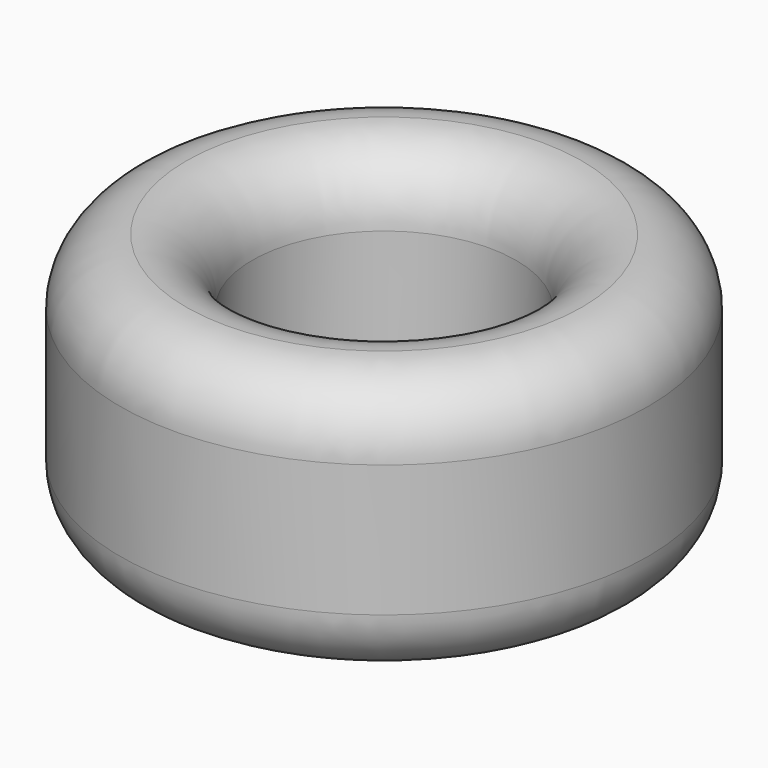
from build123d import *

# Parameters (mm, degrees)
F0_R     = 5.08
F0_R_2   = 2.54
F1_DEPTH = 5.08
F2_R     = 1.26999


# Not quite as in the source:
# - a fillet or chamfer is up to 0.001 mm smaller than in the source, because OpenCascade refuses the exact size


with BuildPart() as f1:
    # F0 (on Top) → F1 (new body)
    with BuildSketch(Plane.XY):
        Circle(F0_R)
        Circle(F0_R_2, mode=Mode.SUBTRACT)
    extrude(amount=F1_DEPTH)

    # F2 (radius 1.27 in the source; OpenCascade refuses exactly that, so slightly less here)
    f2_edges = [f1.edges().sort_by_distance(p)[0] for p in [
        (-5.08, 0, 5.08),
        (-2.54, 0, 5.08),
        (-5.08, 0, 0),
        (-2.54, 0, 0),
    ]]
    fillet(f2_edges, radius=F2_R)


solid = f1.part
